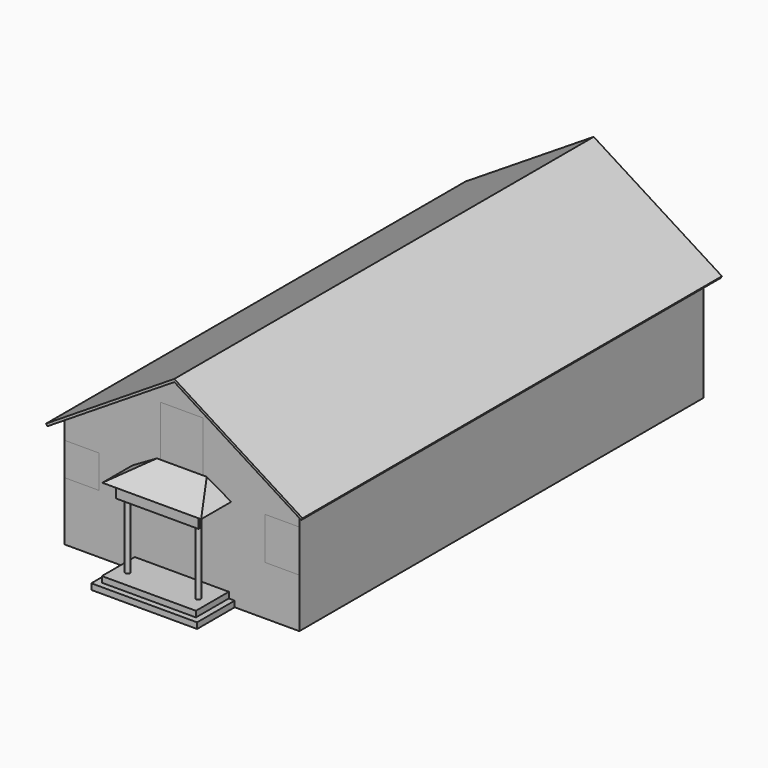
from build123d import *

# Parameters (mm, degrees)
F1_DEPTH  = 10750
F3_DEPTH  = 21500
F5_DEPTH  = 400
F7_DEPTH  = 400
F9_W      = 1800
F9_H      = 2150
F10_DEPTH = 25
F9_W_2    = 1570
F9_H_2    = 1400
F9_W_3    = 1470
F9_H_3    = 1800
F11_R     = 100
F12_DEPTH = 3900
F13_W     = 4200
F13_H     = 1600
F13_R     = 100
F14_DEPTH = 600
F16_DEPTH = 7553.4257402618
F19_DEPTH = 23900.001
F21_DEPTH = 2000
F22_W     = 4000
F22_H     = 250
F23_DEPTH = 250
F24_W     = 3500
F24_H     = 100
F25_DEPTH = 600


with BuildPart() as f1:
    # F0 (on Front) → F1 (new body, symmetric)
    with BuildSketch(Plane.XZ):
        Polygon((0, 7865), (0, 0), (5000, 0), (5000, 4705), align=None)
    extrude(amount=F1_DEPTH, both=True)

    # F2 (on face) → F3 (join)
    with BuildSketch(Plane.XZ.offset(10750)):
        Polygon((5400, 4452.2), (5453.4247402618, 4536.7328168699), (0, 7983.2972527154), (0, 7865), align=None)
    extrude(amount=-F3_DEPTH)

    # F4 (on face) → F5 (join)
    with BuildSketch(Plane.XZ.offset(10750)):
        Polygon((5453.4247402618, 4536.7328168699), (0, 7983.2972527154), (0, 7865), (5000, 4705), (5400, 4452.2), align=None)
    extrude(amount=F5_DEPTH)

    # F6 (on face) → F7 (join)
    with BuildSketch(Plane(origin=(0, 10750, 0), x_dir=(-1, 0, 0), z_dir=(0, 1, 0))):
        Polygon((0, 7865), (0, 7983.2972527154), (-5453.4247402618, 4536.7328168699), (-5400, 4452.2), (-5000, 4705), align=None)
    extrude(amount=F7_DEPTH)

    # F8: F1 across face


with BuildPart() as f1_1:
    add(f1.part)
    add(f1.part.mirror(Plane(origin=(0, 0, 3993.815697783), x_dir=(0, -1, 0), z_dir=(-1, 0, 0))))


with BuildPart() as f10:
    # F9 (on face) → F10 (new body)
    with BuildSketch(Plane.XZ.offset(10750)):
        with Locations((0, 5577)):
            Rectangle(F9_W, F9_H)
    extrude(amount=-F10_DEPTH)


with BuildPart() as f10b:
    # F9 (on face) → F10, piece 2 (new body)
    with BuildSketch(Plane.XZ.offset(10750)):
        with Locations((0, 3200)):
            Rectangle(F9_W_2, F9_H_2)
    extrude(amount=-F10_DEPTH)


with BuildPart() as f10c:
    # F9 (on face) → F10, piece 3 (new body)
    with BuildSketch(Plane.XZ.offset(10750)):
        with Locations((-4265, 3200)):
            Rectangle(F9_W_3, F9_H_2)
    extrude(amount=-F10_DEPTH)


with BuildPart() as f10d:
    # F9 (on face) → F10, piece 4 (new body)
    with BuildSketch(Plane.XZ.offset(10750)):
        with Locations((4265, 3000)):
            Rectangle(F9_W_3, F9_H_3)
    extrude(amount=-F10_DEPTH)


with BuildPart() as f12:
    # F11 (on Top) → F12 (new body)
    with BuildSketch(Plane.XY):
        with Locations((-1500, -11750)):
            Circle(F11_R)
    extrude(amount=F12_DEPTH)


with BuildPart() as f12b:
    # F11 (on Top) → F12, piece 2 (new body)
    with BuildSketch(Plane.XY):
        with Locations((1500, -11750)):
            Circle(F11_R)
    extrude(amount=F12_DEPTH)


with BuildPart() as f14:
    # F13 (on face) → F14 (new body)
    with BuildSketch(Plane.XY.offset(3900)):
        with Locations((0, -11550)):
            Rectangle(F13_W, F13_H)
        with Locations((-1500, -11750)):
            Circle(F13_R, mode=Mode.SUBTRACT)
        with Locations((1500, -11750)):
            Circle(F13_R, mode=Mode.SUBTRACT)
        with Locations((1500, -11750)):
            Circle(F13_R)
        with Locations((-1500, -11750)):
            Circle(F13_R)
    extrude(amount=F14_DEPTH)

    # F15 (on face) → F16 (cut, through all)
    with BuildSketch(Plane.YZ.offset(2100)):
        Polygon((-12350, 4500), (-12350, 3900), (-10750, 4500), align=None)
    extrude(amount=-F16_DEPTH, mode=Mode.SUBTRACT)

    # F18 (on offset) → F19 (cut, through all)
    with BuildSketch(Plane.XZ.offset(12750)):
        Polygon((-2100, 3900), (-1060.7695154587, 4500), (-2100, 4500), align=None)
        Polygon((2100, 3900), (2100, 4500), (1060.7695154587, 4500), align=None)
    extrude(amount=-F19_DEPTH, mode=Mode.SUBTRACT)


with BuildPart() as f21:
    # F20 (on face) → F21 (new body)
    with BuildSketch(Plane.XZ.offset(10750)):
        Polygon((-2250, 250), (-2250, 0), (2250, 0), (2250, 250), (2000, 250), (2000, 500), (-2000, 500), (-2000, 250), align=None)
    extrude(amount=F21_DEPTH)

    # F22 (on face) → F23 (cut)
    with BuildSketch(Plane.XZ.offset(12750)):
        with Locations((0, 375)):
            Rectangle(F22_W, F22_H)
    extrude(amount=-F23_DEPTH, mode=Mode.SUBTRACT)


with BuildPart() as f25:
    # F24 (on face) → F25 (new body)
    with BuildSketch(Plane.XY.offset(3900)):
        with Locations((0, -12000)):
            Rectangle(F24_W, F24_H)
    extrude(amount=-F25_DEPTH)


solid = Compound([f1_1.part, f10.part, f10b.part, f10c.part, f10d.part, f12.part, f12b.part, f14.part, f21.part, f25.part])
